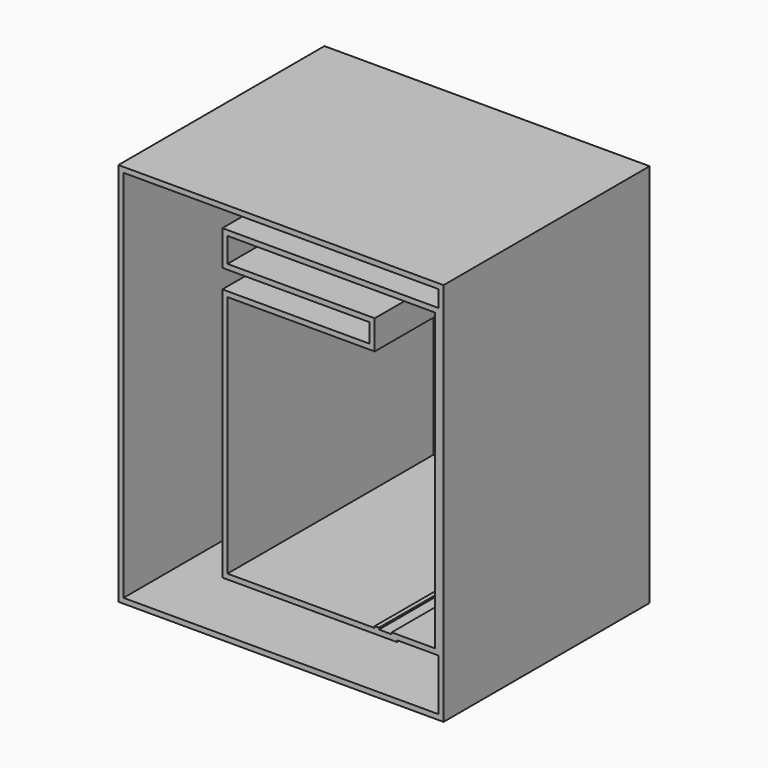
from build123d import *

# Parameters (mm, degrees)
F0_W        = 53.7975355983
F0_H        = 80.8182843029
F0_H_2      = 16.7721658945
F0_H_3      = 21.6287262738
F0_H_4      = 0.8304491639
F0_H_5      = 12.1622607112
F1_DEPTH    = 127
F2_T        = 2.54
F2_T3_DEPTH = 132.08


# Not quite as in the source:
# - a shell that OpenCascade refuses in one call is made with other operations: the cavity is built on its own and cut out


with BuildPart() as f1:
    # F0 (on Front) → F1 (new body)
    with BuildSketch(Plane.XZ):
        with Locations((-143.1119032204, -0.0506583601)):
            Rectangle(F0_W, F0_H)
        with Locations((-143.1119032204, -48.8458834589)):
            Rectangle(F0_W, F0_H_2)
        with Locations((-143.1119032204, -68.046329543)):
            Rectangle(F0_W, F0_H_3)
        Polygon((-170.0106710196, 54.7638610005), (-170.0106710196, 40.3584837914), (-116.2131354213, 40.3584837914), (-74.950940907, 40.3584837914), (-43.6125695705, 40.3584837914), (-43.6125695705, 54.7638610005), (-116.2131354213, 54.7638610005), align=None)
        with Locations((-143.1119032204, -79.2759172618)):
            Rectangle(F0_W, F0_H_4)
        with Locations((-143.1119032204, 60.8449913561)):
            Rectangle(F0_W, F0_H_5)
        Polygon((-116.2131354213, -79.6911418438), (-170.0106710196, -79.6911418438), (-170.0106710196, -109.4150468707), (-9.6626672894, -109.4150468707), (-9.6626672894, -78.8606926799), (-13.8411177322, -78.8606926799), (-35.2556705475, -78.8606926799), (-35.2556705475, -79.6911418438), (-41.5233448148, -79.6911418438), (-41.5233448148, -78.8606926799), (-43.6125695705, -78.8606926799), (-43.6125695705, -79.6911418438), (-74.950940907, -79.6911418438), align=None)
        Polygon((-170.0106710196, 80.1929235458), (-170.0106710196, 66.9261217117), (-116.2131354213, 66.9261217117), (-43.6125695705, 66.9261217117), (-13.8411177322, 66.9261217117), (-9.6626672894, 66.9261217117), (-9.6626672894, 80.1929235458), align=None)
        Polygon((-13.8411177322, 54.7638610005), (-13.8411177322, 40.3584837914), (-13.8411177322, 6.9799921475), (-13.8411177322, -32.6986536384), (-13.8411177322, -78.8606926799), (-9.6626672894, -78.8606926799), (-9.6626672894, 66.9261217117), (-13.8411177322, 66.9261217117), align=None)
    extrude(amount=F1_DEPTH)

    # F2: shell of thickness 2.54, made by hand


with BuildPart() as f2_core1:
    # F2_t2: copy of F1
    add(f1.part)

    # the walls: a layer under each face that stays
    f2_faces = [f2_core1.faces().sort_by_distance(p)[0] for p in [
        (-79.9128524959, -63.5, 40.3584837914),
        (-43.6125695705, -63.5, 47.5611723959),
        (-79.9128524959, -63.5, 54.7638610005),
        (-116.2131354213, -63.5, 60.8449913561),
        (-65.0271265768, -63.5, 66.9261217117),
        (-13.8411177322, -63.5, -5.9672854841),
        (-24.5483941399, -63.5, -78.8606926799),
        (-35.2556705475, -63.5, -79.2759172618),
        (-38.3895076811, -63.5, -79.6911418438),
        (-41.5233448148, -63.5, -79.2759172618),
        (-42.5679571927, -63.5, -78.8606926799),
        (-43.6125695705, -63.5, -79.2759172618),
        (-79.9128524959, -63.5, -79.6911418438),
        (-116.2131354213, -63.5, -19.6663290262),
        (-89.8366691545, -63.5, 80.1929235458),
        (-170.0106710196, -63.5, -14.6110616624),
        (-89.8366691545, -63.5, -109.4150468707),
        (-9.6626672894, -63.5, -14.6110616624),
        (-143.2860037312, 0, -77.813718468),
    ]]
    thicken(f2_faces, amount=-F2_T, mode=Mode.SUBTRACT)

    # F2_s4 → F2_t3 (cut)
    with BuildSketch(Plane.XZ.offset(-2.54)):
        Polygon((-116.1877354213, 40.3330837914), (-116.2131354213, 42.8984837914), (-118.7531354213, 42.8984837914), (-118.7531354213, 40.3584837914), align=None)
        Polygon((-116.1877354213, 54.7892610005), (-116.2131354213, 52.2238610005), (-118.7531354213, 52.2238610005), (-118.7531354213, 54.7638610005), align=None)
        Polygon((-116.1877354213, 66.9007217117), (-118.7531354213, 66.9261217117), (-118.7531354213, 69.4661217117), (-116.2131354213, 69.4661217117), align=None)
        Polygon((-13.8665177322, 66.9007217117), (-13.8411177322, 69.4661217117), (-11.3011177322, 69.4661217117), (-11.3011177322, 66.9261217117), align=None)
        Polygon((-13.8665177322, -78.8352926799), (-11.3011177322, -78.8606926799), (-11.3011177322, -81.4006926799), (-13.8411177322, -81.4006926799), align=None)
        Polygon((-35.2810705475, -79.6657418438), (-32.7156705475, -79.6911418438), (-32.7156705475, -82.2311418438), (-35.2556705475, -82.2311418438), align=None)
        Polygon((-41.4979448148, -79.6657418438), (-41.5233448148, -82.2311418438), (-44.0633448148, -82.2311418438), (-44.0633448148, -79.6911418438), align=None)
        Polygon((-43.6379695705, -79.6657418438), (-41.0725695705, -79.6911418438), (-41.0725695705, -82.2311418438), (-43.6125695705, -82.2311418438), align=None)
        Polygon((-116.1877354213, -79.6657418438), (-116.2131354213, -82.2311418438), (-118.7531354213, -82.2311418438), (-118.7531354213, -79.6911418438), align=None)
    extrude(amount=F2_T3_DEPTH, mode=Mode.SUBTRACT)


with BuildPart() as f1_1:
    add(f1.part)

    # what is left inside the walls is the cavity
    f2_cavity = [f2_core1.part.solids().sort_by_distance(p)[0] for p in [
        (-167.445271, -85.513333, -14.611062),
    ]]
    add(f2_cavity, mode=Mode.SUBTRACT)


solid = f1_1.part
